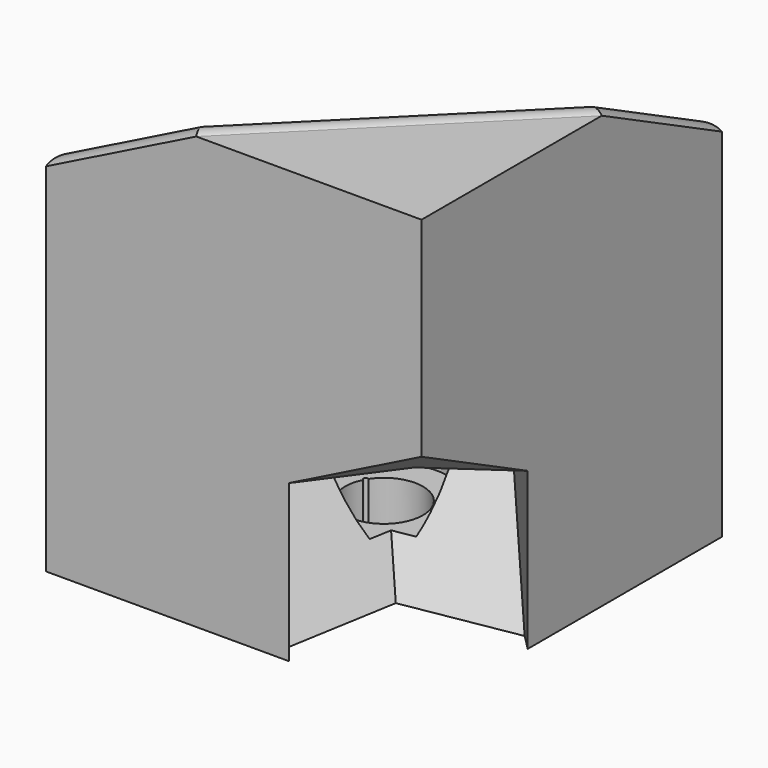
from build123d import *

# Parameters (mm, degrees)
F0_W         = 40
F0_H         = 40
F1_DEPTH     = 20
F3_DEPTH     = 18
F4_DEPTH     = 8
F5_R         = 48.402363322
F6_DEPTH     = 25
F7_R         = 8
F8_DEPTH     = 47.3578016938
F11_DEPTH    = 37.5
F12_DEPTH    = 12.05
F13_R        = 3.85
F14_DEPTH    = 2
F15_DEPTH    = 25
F16_R        = 7
F17_DEPTH    = 13
F18_DEPTH    = 18.5
F19_R        = 1
F20_R        = 11.2
F20_R_2      = 9.2
F21_DEPTH    = 1
F22_T1_DEPTH = 26.5487978578
F22_T3_DEPTH = 53.3816135878
F22_T5_DEPTH = 53.3816135878
F22_T7_DEPTH = 26.5487978578
F22_T9_DEPTH = 42.6013795348


# Not quite as in the source:
# - a fillet or chamfer that OpenCascade refuses, or shapes differently, is made with other operations: its cross-section is extruded or revolved along the edge and cut away or added


with BuildPart() as f1:
    # F0 (on Top) → F1 (new body)
    with BuildSketch(Plane.XY):
        Rectangle(F0_W, F0_H)
    extrude(amount=F1_DEPTH)

    # F3 (add): a face of the model
    f3_faces = [f1.faces().sort_by_distance(p)[0] for p in [
        (0, 0, 0),
    ]]
    extrude(f3_faces, amount=F3_DEPTH)

    # F4 (add): a face of the model
    f4_faces = [f1.faces().sort_by_distance(p)[0] for p in [
        (0, 0, 20),
    ]]
    extrude(f4_faces, amount=F4_DEPTH)

    # F5 (on 3pt) → F6 (cut)
    with BuildSketch(Plane(origin=(-6.6666666667, 6.6666666667, 13.3333333333), x_dir=(0.9128709292, 0.1825741858, 0.3651483717), z_dir=(-0.4082482905, 0.4082482905, 0.8164965809))):
        with Locations((2.3868493736, -7.4885585345)):
            Circle(F5_R)
    extrude(amount=F6_DEPTH, mode=Mode.SUBTRACT)

    # F7 (on face) → F8 (cut, through all)
    with BuildSketch(Plane(origin=(-6.6666666667, 6.6666666667, 13.3333333333), x_dir=(0.9128709292, 0.1825741858, 0.3651483717), z_dir=(-0.4082482905, 0.4082482905, 0.8164965809))):
        with Locations((5.3147843089, -6.5092548249)):
            Circle(F7_R)
    extrude(amount=-F8_DEPTH, mode=Mode.SUBTRACT)

    # F10 (on offset) → F11 (cut, symmetric)
    with BuildSketch(Plane(origin=(9.6632649519, -9.6632649519, -19.3265299038), x_dir=(0.9128709292, 0.1825741858, 0.3651483717), z_dir=(-0.4082482905, 0.4082482905, 0.8164965809))):
        Polygon((16.712234718, -4.6568354596), (9.4092672846, 4.2874364504), (-1.9881831245, 2.4350170851), (-6.0826661002, -8.3616741902), (1.2203013332, -17.3059461002), align=None)
        Polygon((12.6177517423, -15.4535267349), (16.712234718, -4.6568354596), (1.2203013332, -17.3059461002), align=None)
    extrude(amount=F11_DEPTH, both=True, mode=Mode.SUBTRACT)

    # F10 (on offset) → F12 (cut)
    with BuildSketch(Plane(origin=(9.6632649519, -9.6632649519, -19.3265299038), x_dir=(0.9128709292, 0.1825741858, 0.3651483717), z_dir=(-0.4082482905, 0.4082482905, 0.8164965809))):
        Polygon((44.0977028976, 17.7033056762), (16.712234718, -4.6568354596), (12.6177517423, -15.4535267349), (1.2203013332, -17.3059461002), (-18.4589771374, -33.3740096866), (-1.5124044388, -54.1292376868), (61.0442755962, -3.051922324), align=None)
    extrude(amount=F12_DEPTH, mode=Mode.SUBTRACT)

    # F13 (on face) → F14 (join)
    with BuildSketch(Plane(origin=(0, 0, -18), x_dir=(1, 0, 0), z_dir=(0, 0, -1))):
        with Locations((-13.5, 13.5)):
            Circle(F13_R)
        with Locations((-13.5, -13.5)):
            Circle(F13_R)
        with Locations((13.5, -13.5)):
            Circle(F13_R)
    extrude(amount=F14_DEPTH)

    # F13 (on face) → F15 (cut)
    with BuildSketch(Plane(origin=(0, 0, -18), x_dir=(1, 0, 0), z_dir=(0, 0, -1))):
        with BuildLine():
            ThreePointArc((0.2498865688, 4.1424698795), (0, 4.4), (-0.2498865688, 4.1424698795))
            ThreePointArc((-0.2498865688, 4.1424698795), (-3.5940054257, 2.075), (-3.7124274345, -1.8548268231))
            ThreePointArc((-3.7124274345, -1.8548268231), (-3.8105117767, -2.2), (-3.4625408657, -2.2876430564))
            ThreePointArc((-3.4625408657, -2.2876430564), (0, -4.15), (3.4625408657, -2.2876430564))
            ThreePointArc((3.4625408657, -2.2876430564), (3.8105117767, -2.2), (3.7124274345, -1.8548268231))
            ThreePointArc((3.7124274345, -1.8548268231), (3.5940054257, 2.075), (0.2498865688, 4.1424698795))
        make_face()
    extrude(amount=-F15_DEPTH, mode=Mode.SUBTRACT)

    # F16 (on Top) → F17 (cut)
    with BuildSketch(Plane.XY):
        Circle(F16_R)
    extrude(amount=-F17_DEPTH, mode=Mode.SUBTRACT)

    # F16 (on Top) → F18 (cut)
    with BuildSketch(Plane.XY):
        Circle(F16_R)
    extrude(amount=F18_DEPTH, mode=Mode.SUBTRACT)

    # F19
    f19_edges = [f1.edges().sort_by_distance(p)[0] for p in [
        (-17.35, 13.5, -20),
        (-17.35, -13.5, -20),
        (9.65, 13.5, -20),
    ]]
    fillet(f19_edges, radius=F19_R)

    # F20 (on face) → F21 (join)
    with BuildSketch(Plane(origin=(-6.6666666667, 6.6666666667, 13.3333333333), x_dir=(0.9128709292, 0.1825741858, 0.3651483717), z_dir=(-0.4082482905, 0.4082482905, 0.8164965809))):
        Polygon((2.9211869734, -30.410524494), (29.2118697336, -8.94427191), (29.2118697336, 8.94427191), (-14.6059348668, 17.88854382), (-14.6059348668, -26.83281573), align=None)
        Polygon((27.2118697336, -7.9952761744), (2.3913648452, -28.2611335526), (-12.6059348668, -25.1998225681), (-12.6059348668, 15.4390540772), (27.2118697336, 7.3112787481), align=None, mode=Mode.SUBTRACT)
        with Locations((5.3147843089, -6.5092548249)):
            Circle(F20_R)
        with Locations((5.3147843089, -6.5092548249)):
            Circle(F20_R_2, mode=Mode.SUBTRACT)
    extrude(amount=F21_DEPTH)

    # F22: fillet of radius 2 on 5 edges, made by hand

    # F22_s2 → F22_t1 (cut)
    with BuildSketch(Plane(origin=(-11.8729833462, 0, -5.9364916731), x_dir=(0, 1, 0), z_dir=(0.894427191, 0, 0.4472135955))):
        with BuildLine():
            ThreePointArc((-20, 26.83281573), (-19.0328736084, 27.2022251402), (-18.0106128795, 27.038579878))
            Line((-18.0106128795, 27.038579878), (-17.9942829478, 27.0750947152))
            Line((-17.9942829478, 27.0750947152), (-19.5754217779, 27.7822014963))
            Line((-19.5754217779, 27.7822014963), (-19.6282665467, 27.7620165908))
            ThreePointArc((-19.6282665467, 27.7620165908), (-19.8323906919, 27.3055811262), (-20.0234578108, 26.8652152842))
            Line((-20.0234578108, 26.8652152842), (-20, 26.83281573))
        make_face()
    extrude(amount=F22_T1_DEPTH, mode=Mode.SUBTRACT)

    # F22_s4 → F22_t3 (cut)
    with BuildSketch(Plane(origin=(0, 19.8729833462, -9.9364916731), x_dir=(1, 0, 0), z_dir=(0, -0.894427191, 0.4472135955))):
        with BuildLine():
            ThreePointArc((-20, 8.94427191), (-19.6305905898, 9.9113983016), (-18.8271094604, 10.5642496204))
            Line((-18.8271094604, 10.5642496204), (-18.843439392, 10.6007644575))
            Line((-18.843439392, 10.6007644575), (-20.4245782221, 9.8936576763))
            Line((-20.4245782221, 9.8936576763), (-20.4447631276, 9.8408129076))
            ThreePointArc((-20.4447631276, 9.8408129076), (-20.2406389824, 9.384377443), (-20.0397877424, 8.948387193))
            Line((-20.0397877424, 8.948387193), (-20, 8.94427191))
        make_face()
    extrude(amount=F22_T3_DEPTH, mode=Mode.SUBTRACT)

    # F22_s6 → F22_t5 (cut)
    with BuildSketch(Plane(origin=(27.8729833462, 0, 13.9364916731), x_dir=(0, 1, 0), z_dir=(-0.894427191, 0, -0.4472135955))):
        with BuildLine():
            ThreePointArc((20, -8.94427191), (19.6305905898, -9.9113983016), (18.8271094604, -10.5642496204))
            Line((18.8271094604, -10.5642496204), (18.843439392, -10.6007644575))
            Line((18.843439392, -10.6007644575), (20.4245782221, -9.8936576763))
            Line((20.4245782221, -9.8936576763), (20.4447631276, -9.8408129076))
            ThreePointArc((20.4447631276, -9.8408129076), (20.2406389824, -9.384377443), (20.0397877424, -8.948387193))
            Line((20.0397877424, -8.948387193), (20, -8.94427191))
        make_face()
    extrude(amount=F22_T5_DEPTH, mode=Mode.SUBTRACT)

    # F22_s8 → F22_t7 (cut)
    with BuildSketch(Plane(origin=(0, -11.8729833462, 5.9364916731), x_dir=(1, 0, 0), z_dir=(0, 0.894427191, -0.4472135955))):
        with BuildLine():
            ThreePointArc((20, -26.83281573), (19.0328736084, -27.2022251402), (18.0106128795, -27.038579878))
            Line((18.0106128795, -27.038579878), (17.9942829478, -27.0750947152))
            Line((17.9942829478, -27.0750947152), (19.5754217779, -27.7822014963))
            Line((19.5754217779, -27.7822014963), (19.6282665467, -27.7620165908))
            ThreePointArc((19.6282665467, -27.7620165908), (19.8323906919, -27.3055811262), (20.0234578108, -26.8652152842))
            Line((20.0234578108, -26.8652152842), (20, -26.83281573))
        make_face()
    extrude(amount=F22_T7_DEPTH, mode=Mode.SUBTRACT)

    # F22_s10 → F22_t9 (cut)
    with BuildSketch(Plane(origin=(-15.0618621785, -15.0618621785, 0), x_dir=(0, 0, 1), z_dir=(0.7071067812, 0.7071067812, 0))):
        with BuildLine():
            ThreePointArc((27.8164965809, 9.3221446674), (28.1750672506, 10.2933417867), (28, 11.313708499))
            Line((28, 11.313708499), (28.0363299316, 11.3304457648))
            ThreePointArc((28.0363299316, 11.3304457648), (28.4313423012, 11.0576932276), (28.8395905917, 10.769018093))
            Line((28.8395905917, 10.769018093), (28.8491564442, 10.713264219))
            Line((28.8491564442, 10.713264219), (27.8491564442, 9.2990506567))
            Line((27.8491564442, 9.2990506567), (27.8164965809, 9.3221446674))
        make_face()
    extrude(amount=F22_T9_DEPTH, mode=Mode.SUBTRACT)


solid = f1.part
